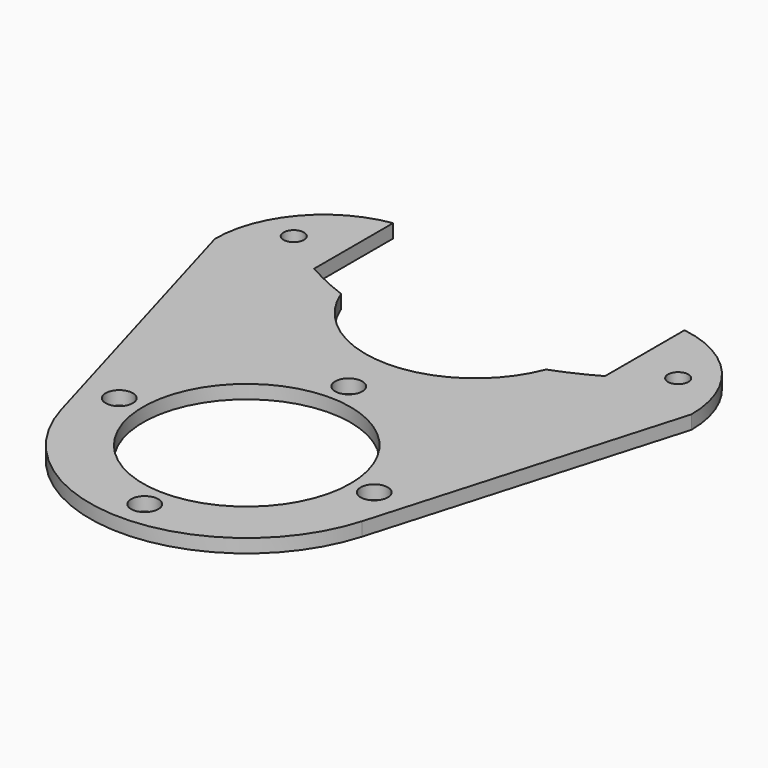
from build123d import *

# Parameters (mm, degrees)
F1_DEPTH = 6.35


# Not quite as in the source:
# - ends of sketch curves that miss each other by under 0.0002 mm in the source are joined


with BuildPart() as f1:
    # F0 (on Top) → F1 (new body)
    with BuildSketch(Plane.XY):
        with BuildLine():
            Line((-111.08563, 71.3839822), (-70.59041, -68.9586378))
            ThreePointArc((-70.59041, -68.9586378), (-0.3347578994, -121.8821648179), (70.0620962947, -69.1465996345))
            Line((70.0620962947, -69.1465996345), (111.08563, 71.6151222))
            ThreePointArc((111.08563, 71.6151222), (98.7152655637, 104.8392134799), (67.6282616967, 121.882228124))
            Line((67.6282616967, 121.882228124), (67.628262, 75.5002554))
            ThreePointArc((67.628262, 75.5002554), (57.7977885358, 70.4247346397), (47.5906584666, 66.156994374))
            ThreePointArc((47.5906584666, 66.156994374), (-0.23749, 33.3973424), (-48.0656463013, 66.1569896482))
            ThreePointArc((-48.0656463013, 66.1569896482), (-58.2727685358, 70.4247346397), (-68.1032374015, 75.5002634895))
            Line((-68.1032374015, 75.5002634895), (-68.103242, 121.5776334))
            ThreePointArc((-68.103242, 121.5776334), (-98.8713942195, 104.4249578962), (-111.08563, 71.3839822))
        make_face()
        with BuildLine():
            ThreePointArc((-6.58749, -108.1531492), (-0.23749, -101.8031492), (6.11251, -108.1531492))
            ThreePointArc((6.11251, -108.1531492), (-0.23749, -114.5031492), (-6.58749, -108.1531492))
        make_face(mode=Mode.SUBTRACT)
        with BuildLine():
            ThreePointArc((-66.0816814, -48.6589578), (-59.7316814, -42.3089578), (-53.3816814, -48.6589578))
            ThreePointArc((-53.3816814, -48.6589578), (-59.7316814, -55.0089578), (-66.0816814, -48.6589578))
        make_face(mode=Mode.SUBTRACT)
        with BuildLine():
            ThreePointArc((-48.65624, -48.6589578), (-0.23749, -0.2402078), (48.18126, -48.6589578))
            ThreePointArc((48.18126, -48.6589578), (-0.23749, -97.0777078), (-48.65624, -48.6589578))
        make_face(mode=Mode.SUBTRACT)
        with BuildLine():
            ThreePointArc((52.9067014, -48.6589578), (59.2567014, -42.3089578), (65.6067014, -48.6589578))
            ThreePointArc((65.6067014, -48.6589578), (59.2567014, -55.0089578), (52.9067014, -48.6589578))
        make_face(mode=Mode.SUBTRACT)
        with BuildLine():
            ThreePointArc((-6.58749, 10.8352336), (-0.23749, 17.1852336), (6.11251, 10.8352336))
            ThreePointArc((6.11251, 10.8352336), (-0.23749, 4.4852336), (-6.58749, 10.8352336))
        make_face(mode=Mode.SUBTRACT)
        with BuildLine():
            ThreePointArc((-94.69374, 90.8966432), (-89.93124, 95.6591432), (-85.16874, 90.8966432))
            ThreePointArc((-85.16874, 90.8966432), (-89.93124, 86.1341432), (-94.69374, 90.8966432))
        make_face(mode=Mode.SUBTRACT)
        with BuildLine():
            ThreePointArc((84.69376, 90.8966432), (89.45626, 95.6591432), (94.21876, 90.8966432))
            ThreePointArc((94.21876, 90.8966432), (89.45626, 86.1341432), (84.69376, 90.8966432))
        make_face(mode=Mode.SUBTRACT)
    extrude(amount=F1_DEPTH)


solid = f1.part
